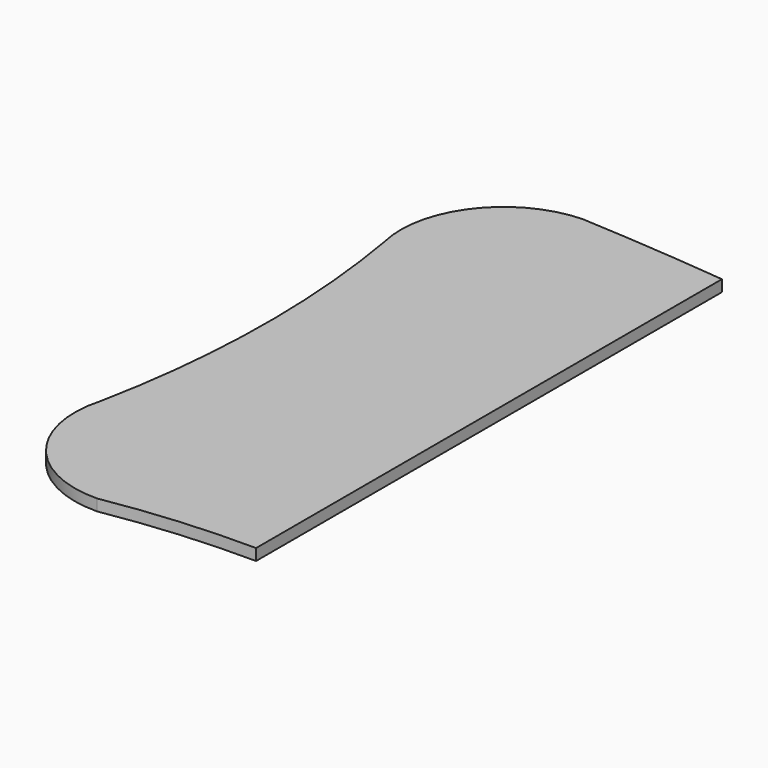
from build123d import *

# Parameters (mm, degrees)
F1_DEPTH = 25.4


# Not quite as in the source:
# - a feature names something its author has since deleted; it is built from what else it names


with BuildPart() as f1:
    # F0 (on Top) → F1 (new body)
    with BuildSketch(Plane.XY):
        with BuildLine():
            Line((-122.74547472, 388.6861801147), (-122.74547472, 642.6861801147))
            ThreePointArc((-122.74547472, 642.6861801147), (-287.6923004816, 657.3774452139), (-452.94547472, 668.0861801147))
            ThreePointArc((-452.94547472, 668.0861801147), (-626.8733109875, 579.3690535942), (-668.84547472, 388.6861801147))
            ThreePointArc((-668.84547472, 388.6861801147), (-637.6124772586, -0.4255791053), (-678.8013792429, -388.6097308259))
            ThreePointArc((-678.8013792429, -388.6097308259), (-639.8991633536, -590.3001733537), (-454.793114458, -679.3404320597))
            ThreePointArc((-454.793114458, -679.3404320597), (-289.3663068571, -658.5539308279), (-122.74547472, -652.5868876355))
            Line((-122.74547472, -652.5868876355), (-122.74547472, 388.6861801147))
        make_face()
    extrude(amount=F1_DEPTH)


solid = f1.part
